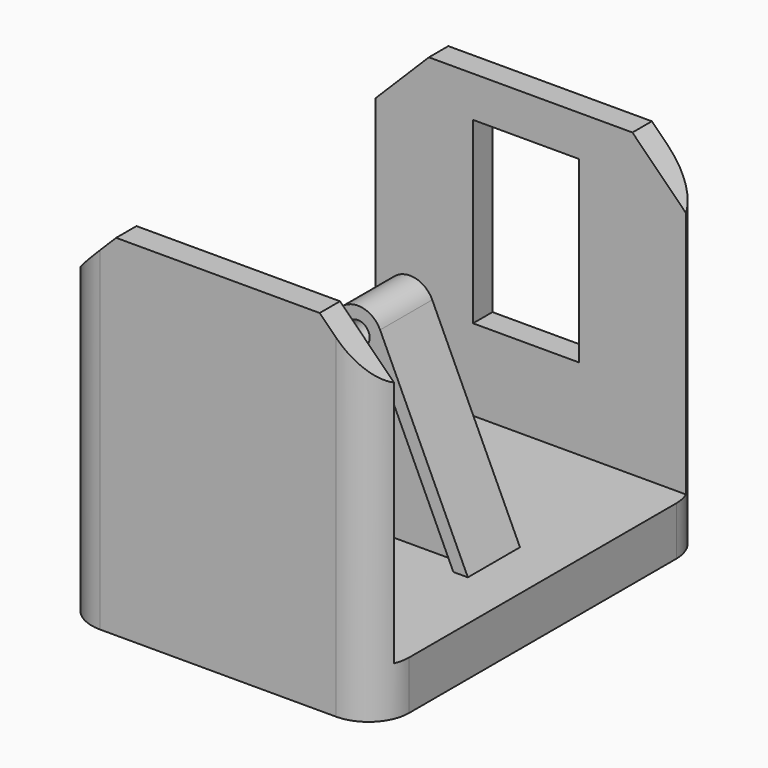
from build123d import *

# Parameters (mm, degrees)
F0_W          = 39
F0_H          = 51
F1_DEPTH      = 6
F2_R          = 1.4383077573
F3_DEPTH      = 4
F3_DEPTH_BACK = 4
F5_DEPTH      = 2
F6_W          = 39
F6_H          = 2.9835407734
F6_H_2        = 3.1214025915
F7_DEPTH      = 37
F8_SIZE       = 7
F9_T1_DEPTH   = 61
F10_W         = 13
F10_H         = 22
F11_DEPTH     = 15.8


# Not quite as in the source:
# - a fillet or chamfer that OpenCascade refuses, or shapes differently, is made with other operations: its cross-section is extruded or revolved along the edge and cut away or added
# - a pattern or mirror of a feature is missing from the dataset's text; its kind, count and spacing are read off the source's solid


with BuildPart() as f1:
    # F0 (on Top) → F1 (new body)
    with BuildSketch(Plane.XY):
        Rectangle(F0_W, F0_H)
    extrude(amount=F1_DEPTH)

    # F2 (on Front) → F3 (join, two sides)
    with BuildSketch(Plane.XZ) as f3_sk:
        with BuildLine():
            Line((-2.7218379916, 29.2536051472), (-13.5, 6))
            Line((-13.5, 6), (13.5, 6))
            Line((13.5, 6), (2.7218379916, 29.2536051472))
            ThreePointArc((2.7218379916, 29.2536051472), (0, 30.9920196576), (-2.7218379916, 29.2536051472))
        make_face()
        with Locations((0, 27.9920196576)):
            Circle(F2_R, mode=Mode.SUBTRACT)
    extrude(amount=F3_DEPTH)
    extrude(f3_sk.sketch, amount=-F3_DEPTH_BACK)

    # F4 (on face) → F5 (cut)
    with BuildSketch(Plane.XZ.offset(4)):
        with BuildLine():
            Line((-2.3500163027, 26.2716104284), (-11.7460088804, 6))
            Line((-11.7460088804, 6), (11.7170447484, 6))
            Line((11.7170447484, 6), (2.3322070272, 26.2475441144))
            ThreePointArc((2.3322070272, 26.2475441144), (-0.0149696172, 25.0796047749), (-2.3500163027, 26.2716104284))
        make_face()
    f5 = extrude(amount=-F5_DEPTH, mode=Mode.SUBTRACT)

    # F5_copies: F5 across plane
    add(f5.mirror(Plane.ZX), mode=Mode.SUBTRACT)

    # F6 (on face) → F7 (join)
    with BuildSketch(Plane.XY.offset(6)):
        with Locations((0, 24.0082296133)):
            Rectangle(F6_W, F6_H)
        with Locations((0, -23.9392987043)):
            Rectangle(F6_W, F6_H_2)
    extrude(amount=F7_DEPTH)

    # F8
    f8_edges = [f1.edges().sort_by_distance(p)[0] for p in [
        (19.5, 24.00823, 43),
        (-19.5, 24.00823, 43),
        (-19.5, -23.939299, 43),
        (19.5, -23.939299, 43),
    ]]
    chamfer(f8_edges, length=F8_SIZE)

    # F9: fillet of radius 5 on 4 edges, made by hand

    # F9_s2 → F9_t1 (cut)
    with BuildSketch(Plane.XY.offset(-12.5)):
        with BuildLine():
            ThreePointArc((19.5, -20.5), (18.0355339059, -24.0355339059), (14.5, -25.5))
            Line((14.5, -25.5), (19.5, -25.5))
            Line((19.5, -25.5), (19.5, -20.5))
        make_face()
        with BuildLine():
            ThreePointArc((-19.5, -20.5), (-18.0355339059, -24.0355339059), (-14.5, -25.5))
            Line((-14.5, -25.5), (-19.5, -25.5))
            Line((-19.5, -25.5), (-19.5, -20.5))
        make_face()
        with BuildLine():
            ThreePointArc((14.5, 25.5), (18.0355339059, 24.0355339059), (19.5, 20.5))
            Line((19.5, 20.5), (19.5, 25.5))
            Line((19.5, 25.5), (14.5, 25.5))
        make_face()
        with BuildLine():
            ThreePointArc((-14.5, 25.5), (-18.0355339059, 24.0355339059), (-19.5, 20.5))
            Line((-19.5, 20.5), (-19.5, 25.5))
            Line((-19.5, 25.5), (-14.5, 25.5))
        make_face()
    extrude(amount=F9_T1_DEPTH, mode=Mode.SUBTRACT)

    # F10 (on face) → F11 (cut)
    with BuildSketch(Plane(origin=(0, 25.5, 0), x_dir=(-1, 0, 0), z_dir=(0, 1, 0))):
        with Locations((0.5753570557, 27)):
            Rectangle(F10_W, F10_H)
    extrude(amount=-F11_DEPTH, mode=Mode.SUBTRACT)


solid = f1.part
